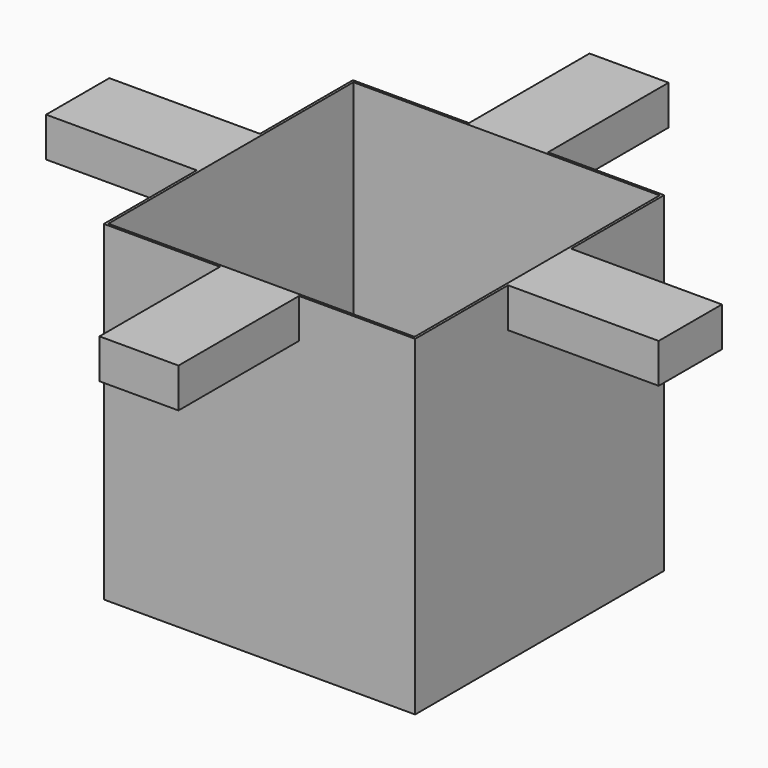
from build123d import *

# Parameters (mm, degrees)
F0_W      = 40
F0_H      = 42.5
F1_DEPTH  = 20
F2_W      = 39.365
F2_H      = 39.365
F3_DEPTH  = 41.865
F4_W      = 10.16
F4_H      = 5.08
F8_DEPTH  = 19.365
F5_W      = 10.16
F5_H      = 5.08
F9_DEPTH  = 19.365
F6_W      = 10.16
F6_H      = 5.08
F10_DEPTH = 19.365
F7_W      = 10.16
F7_H      = 5.08
F11_DEPTH = 19.365


with BuildPart() as f1:
    # F0 (on Front) → F1 (new body, symmetric)
    with BuildSketch(Plane.XZ):
        Rectangle(F0_W, F0_H)
    extrude(amount=F1_DEPTH, both=True)

    # F2 (on face) → F3 (cut)
    with BuildSketch(Plane.XY.offset(21.25)):
        Rectangle(F2_W, F2_H)
    extrude(amount=-F3_DEPTH, mode=Mode.SUBTRACT)

    # F4 (on face) → F8 (join)
    with BuildSketch(Plane.XZ.offset(20)):
        with Locations((0, 18.71)):
            Rectangle(F4_W, F4_H)
    extrude(amount=F8_DEPTH)

    # F5 (on face) → F9 (join)
    with BuildSketch(Plane(origin=(-20, 0, 0), x_dir=(0, -1, 0), z_dir=(-1, 0, 0))):
        with Locations((0, 18.71)):
            Rectangle(F5_W, F5_H)
    extrude(amount=F9_DEPTH)

    # F6 (on face) → F10 (join)
    with BuildSketch(Plane(origin=(0, 20, 0), x_dir=(-1, 0, 0), z_dir=(0, 1, 0))):
        with Locations((0, 18.71)):
            Rectangle(F6_W, F6_H)
    extrude(amount=F10_DEPTH)

    # F7 (on face) → F11 (join)
    with BuildSketch(Plane.YZ.offset(20)):
        with Locations((0, 18.71)):
            Rectangle(F7_W, F7_H)
    extrude(amount=F11_DEPTH)


solid = f1.part
